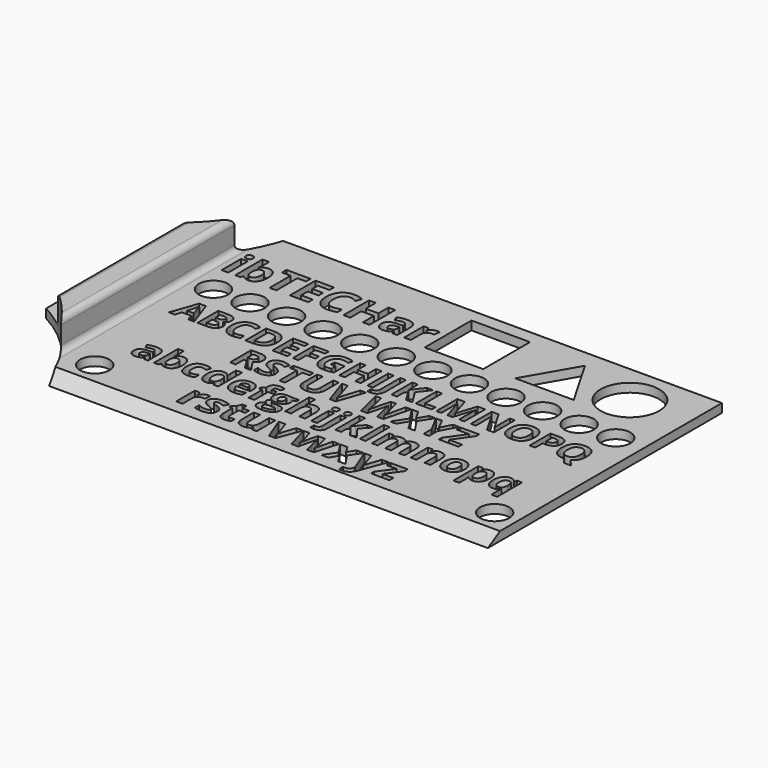
from build123d import *

# Parameters (mm, degrees)
F1_DEPTH       = 3
F3_DEPTH       = 10
F4_T4_DEPTH    = 84.0416899581
F4_S5_R        = 52
F4_T6_DEPTH    = 44
F4_S7_R        = 52
F4_T8_DEPTH    = 44
F4_T12_DEPTH   = 61.7868841557
F4_S13_R       = 52
F4_T14_DEPTH   = 32
F4_S15_R       = 52
F4_T16_DEPTH   = 32
F4_T17_DEPTH   = 84.0416899581
F4_T19_DEPTH   = 61.7868841557
F5_W           = 20
F5_H           = 20
F5_R           = 10
F5_R_2         = 5
F5_TEXT_SIZE   = 15.2791514614
F5_TEXT_SIZE_2 = 12.4876308344
F5_TEXT_SIZE_3 = 12.6310595781
F5_TEXT_SIZE_4 = 13.4983857099
F5_TEXT_SIZE_5 = 14.5998722511
F6_DEPTH       = 25
F7_SIZE2       = 5.196142
F7_SIZE        = 2.99999


# Not quite as in the source:
# - a fillet or chamfer that OpenCascade refuses, or shapes differently, is made with other operations: its cross-section is extruded or revolved along the edge and cut away or added
# - a fillet or chamfer is up to 0.001 mm smaller than in the source, because OpenCascade refuses the exact size
# - Text() gives the source's letters only with a copy of the font that has no kerning and outlines rounded to 1/6400 em; it was checked with that copy


with BuildPart() as f1:
    # F0 (on Top) → F1 (new body)
    with BuildSketch(Plane.XY):
        with BuildLine():
            Line((-62.5, -50), (87.5, -50))
            Line((87.5, -50), (87.5, 50))
            Line((87.5, 50), (-62.5, 50))
            ThreePointArc((-62.5, 50), (-72.0768540724, 32.5640450603), (-87.5, 20))
            Line((-87.5, 20), (-87.5, -20))
            ThreePointArc((-87.5, -20), (-72.0768540724, -32.5640450603), (-62.5, -50))
        make_face()
    extrude(amount=F1_DEPTH)

    # F2 (on face) → F3 (join)
    with BuildSketch(Plane.XY.offset(3)):
        with BuildLine():
            Line((-68.75, 0), (-68.75, 37.020844979))
            ThreePointArc((-68.75, 37.020844979), (-73.3477338965, 31.0956341025), (-78.75, 25.8934420779))
            Line((-78.75, 25.8934420779), (-78.75, 0))
            Line((-78.75, 0), (-78.75, -25.8934420779))
            ThreePointArc((-78.75, -25.8934420779), (-73.3477338965, -31.0956341025), (-68.75, -37.020844979))
            Line((-68.75, -37.020844979), (-68.75, 0))
        make_face()
    extrude(amount=F3_DEPTH)

    # F4: fillet of radius 2 on 4 edges, made by hand


with BuildPart() as f4_tool2:
    # F4_s3 → F4_t4 (new body)
    with BuildSketch(Plane.XZ.offset(42.020844979)):
        with BuildLine():
            ThreePointArc((-66.75, 3), (-68.1642135624, 3.5857864376), (-68.75, 5))
            Line((-68.75, 5), (-68.75, 3))
            Line((-68.75, 3), (-66.75, 3))
        make_face()
    extrude(amount=-F4_T4_DEPTH)

    # F4_s5 → F4_t6 (cut, symmetric)
    with BuildSketch(Plane.XY.offset(4)):
        with Locations((-112.0243606115, -65.8536338429)):
            Circle(F4_S5_R)
    extrude(amount=F4_T6_DEPTH, both=True, mode=Mode.SUBTRACT)

    # F4_s7 → F4_t8 (cut, symmetric)
    with BuildSketch(Plane.XY.offset(4)):
        with Locations((-112.0243606115, 65.8536338429)):
            Circle(F4_S7_R)
    extrude(amount=F4_T8_DEPTH, both=True, mode=Mode.SUBTRACT)


with BuildPart() as f1_1:
    add(f1.part)

    # F4_t1: union F4_tool2
    add(f4_tool2.part)


with BuildPart() as f4_tool10:
    # F4_s11 → F4_t12 (new body)
    with BuildSketch(Plane.XZ.offset(-30.8934420779)):
        with BuildLine():
            ThreePointArc((-80.75, 3), (-79.3357864376, 3.5857864376), (-78.75, 5))
            Line((-78.75, 5), (-78.75, 3))
            Line((-78.75, 3), (-80.75, 3))
        make_face()
    extrude(amount=F4_T12_DEPTH)

    # F4_s13 → F4_t14 (cut, symmetric)
    with BuildSketch(Plane.XY.offset(4)):
        with Locations((-112.0243606115, -65.8536338429)):
            Circle(F4_S13_R)
    extrude(amount=F4_T14_DEPTH, both=True, mode=Mode.SUBTRACT)

    # F4_s15 → F4_t16 (cut, symmetric)
    with BuildSketch(Plane.XY.offset(4)):
        with Locations((-112.0243606115, 65.8536338429)):
            Circle(F4_S15_R)
    extrude(amount=F4_T16_DEPTH, both=True, mode=Mode.SUBTRACT)


with BuildPart() as f1_2:
    add(f1_1.part)

    # F4_t9: union F4_tool10
    add(f4_tool10.part)

    # F4_s18 → F4_t17 (cut)
    with BuildSketch(Plane.XZ.offset(-42.020844979)):
        with BuildLine():
            ThreePointArc((-70.75, 13), (-69.3357864376, 12.4142135624), (-68.75, 11))
            Line((-68.75, 11), (-68.75, 13))
            Line((-68.75, 13), (-70.75, 13))
        make_face()
    extrude(amount=F4_T17_DEPTH, mode=Mode.SUBTRACT)

    # F4_s20 → F4_t19 (cut)
    with BuildSketch(Plane.XZ.offset(-30.8934420779)):
        with BuildLine():
            ThreePointArc((-78.75, 11), (-78.1642135624, 12.4142135624), (-76.75, 13))
            Line((-76.75, 13), (-78.75, 13))
            Line((-78.75, 13), (-78.75, 11))
        make_face()
    extrude(amount=F4_T19_DEPTH, mode=Mode.SUBTRACT)

    # F5 (on face) → F6 (cut)
    with BuildSketch(Plane.XY.offset(3)):
        with Locations((15.5, 35.5)):
            Rectangle(F5_W, F5_H)
        Polygon((45.5, 44), (35.5, 26.6794919243), (55.5, 26.6794919243), align=None)
        with Locations((67.2527924006, 36)):
            Circle(F5_R)
        with Locations((-59.556286782, 16.5726331281)):
            Circle(F5_R_2)
        with Locations((-47.056286782, 16.5726331281)):
            Circle(F5_R_2)
        with Locations((-34.556286782, 16.5726331281)):
            Circle(F5_R_2)
        with Locations((-22.056286782, 16.5726331281)):
            Circle(F5_R_2)
        with Locations((-9.556286782, 16.5726331281)):
            Circle(F5_R_2)
        with Locations((2.943713218, 16.5726331281)):
            Circle(F5_R_2)
        with Locations((15.443713218, 16.5726331281)):
            Circle(F5_R_2)
        with Locations((27.943713218, 16.5726331281)):
            Circle(F5_R_2)
        with Locations((40.443713218, 16.5726331281)):
            Circle(F5_R_2)
        with Locations((52.943713218, 16.5726331281)):
            Circle(F5_R_2)
        with Locations((65.443713218, 16.5726331281)):
            Circle(F5_R_2)
        with Locations((77.943713218, 16.5726331281)):
            Circle(F5_R_2)
        with Locations((79.7107368708, -37.375087738)):
            Circle(F5_R_2)
        with Locations((-56.9626055658, -37.375087738)):
            Circle(F5_R_2)
        with Locations((-65.9527933431, 26.5710618959)):
            Text('ibTECHar', F5_TEXT_SIZE, font='Open Sans', font_style=FontStyle.BOLD, text_align=(TextAlign.LEFT, TextAlign.BOTTOM))
        with Locations((-60.4890270019, -1.2526484364)):
            Text('ABCDEFGHIJKLMNOPQ', F5_TEXT_SIZE_2, font='Open Sans', font_style=FontStyle.BOLD, text_align=(TextAlign.LEFT, TextAlign.BOTTOM))
        with Locations((-30.821820721, -13.654621024)):
            Text('RSTUV WXYZ', F5_TEXT_SIZE_3, font='Open Sans', font_style=FontStyle.BOLD, text_align=(TextAlign.LEFT, TextAlign.BOTTOM))
        with Locations((-54.6025000513, -26.5329735457)):
            Text('abcdefghijklmnopq', F5_TEXT_SIZE_4, font='Open Sans', font_style=FontStyle.BOLD, text_align=(TextAlign.LEFT, TextAlign.BOTTOM))
        with Locations((-27.9626809061, -40.2714257799)):
            Text('rstuvwxyz', F5_TEXT_SIZE_5, font='Open Sans', font_style=FontStyle.BOLD, text_align=(TextAlign.LEFT, TextAlign.BOTTOM))
    extrude(amount=-F6_DEPTH, mode=Mode.SUBTRACT)

    # F7 (size 3 and 5.1961524227 in the source; OpenCascade refuses exactly that, so slightly less here)
    f7_edges = [f1_2.edges().sort_by_distance(p)[0] for p in [
        (12.5, -50, 3),
    ]]
    f7_side = f1_2.faces().sort_by_distance((12.5, -50, 1.5))[0]
    chamfer(f7_edges, length=F7_SIZE, length2=F7_SIZE2, reference=f7_side)


solid = f1_2.part
